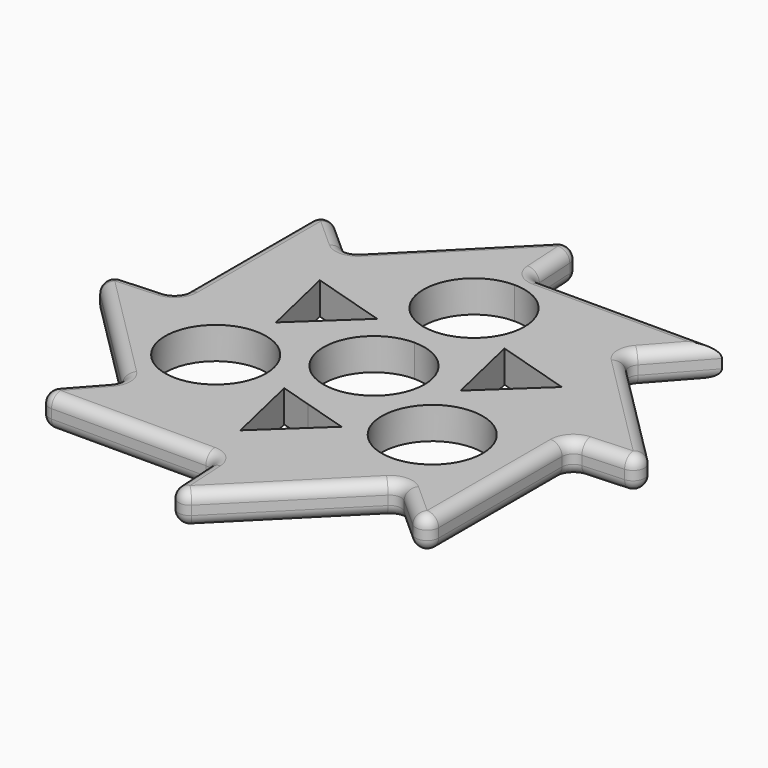
from build123d import *

# Parameters (mm, degrees)
F0_R     = 11.05
F1_DEPTH = 7
F2_F1_R  = 2.5
F2_F2_R  = 2.5


with BuildPart() as f1:
    # F0 (on Top) → F1 (new body)
    with BuildSketch(Plane.XY):
        Polygon((-30.4590901453, -30.4590901453), (0, -43.075658381), (30.4590901453, -30.4590901453), (43.075658381, 0), (30.4590901453, 30.4590901453), (0, 43.075658381), (-30.4590901453, 30.4590901453), (-43.075658381, 0), align=None)
        with Locations((-23.7159928866, -13.6924348772)):
            Circle(F0_R, mode=Mode.SUBTRACT)
        with BuildLine():
            ThreePointArc((0, 11.05), (7.8135299321, 7.8135299321), (11.05, 0))
            ThreePointArc((11.05, 0), (7.8135299321, -7.8135299321), (0, -11.05))
            ThreePointArc((0, -11.05), (-11.05, 0), (0, 11.05))
        make_face(mode=Mode.SUBTRACT)
        Polygon((-6.8369439754, -16.0300867214), (0, -18.1124230949), (9.7544447129, -21.0833462298), (0, -30.1988758228), (-2.9175007375, -32.9252805637), align=None, mode=Mode.SUBTRACT)
        with Locations((23.7159928866, -13.6924348772)):
            Circle(F0_R, mode=Mode.SUBTRACT)
        Polygon((-27.0553790261, 18.989270036), (-10.4639903379, 13.9360105276), (-23.1359357882, 2.0940761937), align=None, mode=Mode.SUBTRACT)
        with BuildLine():
            ThreePointArc((11.05, 27.3848697543), (7.8135299321, 19.5713398222), (0, 16.3348697543))
            ThreePointArc((0, 16.3348697543), (-11.05, 27.3848697543), (0, 38.4348697543))
            ThreePointArc((0, 38.4348697543), (7.8135299321, 35.1983996864), (11.05, 27.3848697543))
        make_face(mode=Mode.SUBTRACT)
        Polygon((13.3814910753, 18.989270036), (29.9728797636, 13.9360105276), (17.3009343133, 2.0940761937), align=None, mode=Mode.SUBTRACT)
        Polygon((-0.9420321136, 59.9761481769), (-30.4590901453, 30.4590901453), (0, 43.075658381), align=None)
        Polygon((-43.075658381, 41.7434237897), (-43.075658381, 0), (-30.4590901453, 30.4590901453), align=None)
        Polygon((-59.9761481769, -0.9420321136), (-30.4590901453, -30.4590901453), (-43.075658381, 0), align=None)
        Polygon((0, 43.075658381), (30.4590901453, 30.4590901453), (41.7434237897, 43.075658381), align=None)
        Polygon((-41.7434237897, -43.075658381), (0, -43.075658381), (-30.4590901453, -30.4590901453), align=None)
        Polygon((30.4590901453, -30.4590901453), (0, -43.075658381), (0.9420321136, -59.9761481769), align=None)
        Polygon((43.075658381, 0), (30.4590901453, -30.4590901453), (43.075658381, -41.7434237897), align=None)
        Polygon((30.4590901453, 30.4590901453), (43.075658381, 0), (59.9761481769, 0.9420321136), align=None)
    extrude(amount=F1_DEPTH)

    # F2: fillet of radius 2.5 on 31 edges, made by hand

    # F2_f1
    f2_f1_edges = [f1.edges().sort_by_distance(p)[0] for p in [
        (-30.4590901453, 30.4590901453, 3.5),
        (0, 43.075658381, 3.5),
        (30.4590901453, 30.4590901453, 3.5),
        (43.075658381, 0, 3.5),
        (30.4590901453, -30.4590901453, 3.5),
        (0, -43.075658381, 3.5),
        (-30.4590901453, -30.4590901453, 3.5),
        (-43.075658381, 0, 3.5),
    ]]
    fillet(f2_f1_edges, radius=F2_F1_R)

    # F2_f2
    f2_f2_edges = [f1.edges().sort_by_distance(p)[0] for p in [
        (-43.075658381, 41.7434237897, 3.5),
        (-37.6485921809, 36.8894235126, 0),
        (-37.6485921809, 36.8894235126, 7),
        (-0.9420321136, 59.9761481769, 3.5),
        (-0.5368133134, 52.7063363531, 0),
        (-0.5368133134, 52.7063363531, 7),
        (59.9761481769, 0.9420321136, 3.5),
        (46.0536070562, 14.8645732343, 0),
        (46.0536070562, 14.8645732343, 7),
        (43.075658381, -41.7434237897, 3.5),
        (43.075658381, -22.0539773141, 0),
        (43.075658381, -22.0539773141, 7),
        (0.9420321136, -59.9761481769, 3.5),
        (14.8645732343, -46.0536070562, 0),
        (14.8645732343, -46.0536070562, 7),
        (-41.7434237897, -43.075658381, 3.5),
        (-22.0539773141, -43.075658381, 0),
        (-22.0539773141, -43.075658381, 7),
        (-59.9761481769, -0.9420321136, 3.5),
        (-46.0536070562, -14.8645732343, 0),
        (-46.0536070562, -14.8645732343, 7),
        (-43.075658381, 22.0539773141, 0),
        (-43.075658381, 22.0539773141, 7),
        (-43.7593661923, 0.6466592818, 7),
        (-43.7593661923, 0.6466592818, 0),
        (-31.3998017383, -30.4852874118, 7),
        (-31.3998017383, -30.4852874118, 0),
        (-0.6466592818, -43.7593661923, 7),
        (-0.6466592818, -43.7593661923, 0),
        (30.4852874118, -31.3998017383, 7),
        (30.4852874118, -31.3998017383, 0),
        (43.7593661923, -0.6466592818, 7),
        (43.7593661923, -0.6466592818, 0),
        (31.3998017383, 30.4852874118, 7),
        (31.3998017383, 30.4852874118, 0),
        (0.6466592818, 43.7593661923, 7),
        (0.6466592818, 43.7593661923, 0),
        (-30.4852874118, 31.3998017383, 7),
        (-30.4852874118, 31.3998017383, 0),
    ]]
    fillet(f2_f2_edges, radius=F2_F2_R)


solid = f1.part
